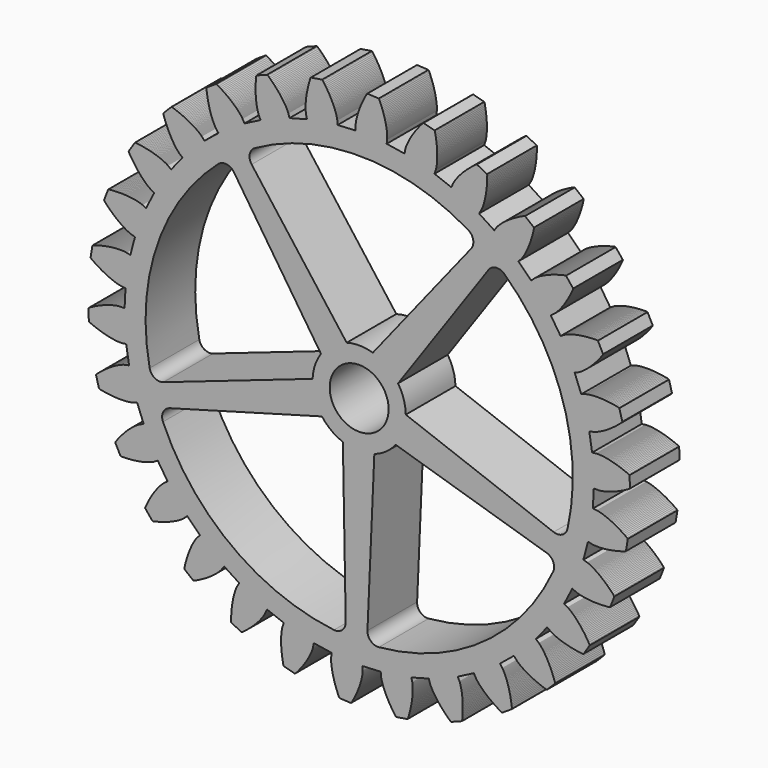
from build123d import *

# Parameters (mm, degrees)
F0_R     = 3.797782
F1_DEPTH = 8


# Not quite as in the source:
# - ends of sketch curves that miss each other by under 0.0002 mm in the source are joined


with BuildPart() as f1:
    # F0 (on Front) → F1 (new body)
    with BuildSketch(Plane.XZ):
        Polygon((-30.117293, 2.712268), (-30.236686, 0.387787), (-30.777096, 0.394663), (-30.78543, 0.394573), (-30.797925, 0.394291), (-30.814581, 0.393725), (-30.835394, 0.392777), (-30.86035, 0.391351), (-30.889447, 0.389347), (-30.92267, 0.386671), (-30.96001, 0.383226), (-31.001451, 0.378913), (-31.04698, 0.373644), (-31.096573, 0.367317), (-31.15022, 0.35984), (-31.207894, 0.351114), (-31.269576, 0.341048), (-31.335238, 0.329545), (-31.404858, 0.316515), (-31.478408, 0.301861), (-31.555862, 0.285489), (-31.637181, 0.26731), (-31.722344, 0.247231), (-31.811308, 0.225156), (-31.904043, 0.200998), (-32.000506, 0.174668), (-32.100667, 0.146072), (-32.204481, 0.115122), (-32.311902, 0.08173), (-32.422897, 0.045809), (-32.537413, 0.00727), (-32.655406, -0.033976), (-32.776828, -0.07801), (-32.901628, -0.12492), (-33.029758, -0.17479), (-33.161166, -0.227706), (-33.295794, -0.283746), (-33.433588, -0.342994), (-33.574489, -0.405532), (-33.718444, -0.471442), (-33.865391, -0.540798), (-34.015269, -0.613683), (-34.168013, -0.69017), (-34.323558, -0.770338), (-34.481844, -0.854264), (-34.6428, -0.942018), (-34.80636, -1.033678), (-34.915142, -1.127462), (-34.836389, -2.600837), (-34.718226, -2.682489), (-34.545831, -2.756192), (-34.376436, -2.826287), (-34.210107, -2.892861), (-34.046901, -2.955992), (-33.886875, -3.015765), (-33.730082, -3.072257), (-33.576582, -3.125552), (-33.426419, -3.175739), (-33.279653, -3.222902), (-33.136328, -3.267125), (-32.996493, -3.308494), (-32.860193, -3.347102), (-32.727478, -3.383027), (-32.598389, -3.416368), (-32.472965, -3.447208), (-32.351247, -3.475639), (-32.233276, -3.501753), (-32.119085, -3.52564), (-32.008712, -3.547388), (-31.902195, -3.567096), (-31.799556, -3.584851), (-31.700834, -3.600751), (-31.606052, -3.614884), (-31.515241, -3.627348), (-31.428425, -3.638238), (-31.345629, -3.647646), (-31.266877, -3.655665), (-31.192182, -3.662397), (-31.12157, -3.667931), (-31.055053, -3.67237), (-30.992651, -3.675804), (-30.934374, -3.67833), (-30.880239, -3.680046), (-30.830252, -3.68105), (-30.784423, -3.681442), (-30.742756, -3.681311), (-30.705264, -3.680754), (-30.671943, -3.679874), (-30.642798, -3.678764), (-30.617832, -3.677525), (-30.597037, -3.67625), (-30.580416, -3.675038), (-30.567963, -3.673983), (-30.559666, -3.673185), (-30.023068, -3.608741), (-29.656569, -5.907251), (-30.186598, -6.012883), (-30.194731, -6.014705), (-30.206896, -6.017575), (-30.223069, -6.021593), (-30.24323, -6.026847), (-30.267345, -6.033432), (-30.295389, -6.041444), (-30.327331, -6.050968), (-30.363138, -6.0621), (-30.402776, -6.074932), (-30.446213, -6.089552), (-30.493409, -6.106054), (-30.544327, -6.124522), (-30.598927, -6.145049), (-30.657167, -6.167716), (-30.719006, -6.192621), (-30.784395, -6.219842), (-30.853291, -6.249467), (-30.925647, -6.281584), (-31.00141, -6.316276), (-31.080535, -6.353622), (-31.162967, -6.393712), (-31.248651, -6.436619), (-31.337534, -6.482434), (-31.429559, -6.531227), (-31.52467, -6.583083), (-31.622805, -6.638081), (-31.723902, -6.696296), (-31.827901, -6.757801), (-31.934741, -6.822677), (-32.044356, -6.890995), (-32.156676, -6.962829), (-32.271639, -7.038248), (-32.389171, -7.117325), (-32.509204, -7.200134), (-32.63167, -7.286737), (-32.756491, -7.377204), (-32.8836, -7.471601), (-33.012915, -7.569996), (-33.144362, -7.672447), (-33.277866, -7.779019), (-33.413347, -7.889777), (-33.550722, -8.004778), (-33.689915, -8.12408), (-33.830841, -8.247742), (-33.91775, -8.362093), (-33.534386, -9.786899), (-33.401831, -9.842198), (-33.217875, -9.878447), (-33.03761, -9.911795), (-32.861075, -9.942331), (-32.68831, -9.97015), (-32.519351, -9.995342), (-32.354241, -10.018002), (-32.193013, -10.038218), (-32.035698, -10.056088), (-31.882334, -10.071706), (-31.732945, -10.085164), (-31.587564, -10.096556), (-31.446219, -10.105981), (-31.308935, -10.113529), (-31.175732, -10.119302), (-31.046637, -10.123391), (-30.921668, -10.125895), (-30.800844, -10.12691), (-30.684184, -10.126533), (-30.571702, -10.124861), (-30.463411, -10.121988), (-30.359328, -10.118017), (-30.259457, -10.113042), (-30.163809, -10.107162), (-30.072389, -10.100474), (-29.985208, -10.093073), (-29.902264, -10.085061), (-29.823564, -10.076532), (-29.749101, -10.067586), (-29.678882, -10.05832), (-29.612897, -10.04883), (-29.551143, -10.039216), (-29.493617, -10.029572), (-29.440304, -10.019994), (-29.391202, -10.010585), (-29.346292, -10.001433), (-29.305566, -9.992644), (-29.269008, -9.984306), (-29.236598, -9.976517), (-29.208323, -9.969373), (-29.184157, -9.962968), (-29.164084, -9.957396), (-29.148077, -9.952753), (-29.136115, -9.949134), (-29.128167, -9.946629), (-28.616692, -9.77203), (-27.780316, -11.94411), (-28.276802, -12.157635), (-28.284376, -12.161104), (-28.295679, -12.166445), (-28.310665, -12.173734), (-28.32929, -12.183066), (-28.351509, -12.194522), (-28.377274, -12.208187), (-28.40654, -12.224146), (-28.439249, -12.24248), (-28.475354, -12.263274), (-28.514803, -12.286605), (-28.557537, -12.312557), (-28.603499, -12.34121), (-28.652639, -12.372638), (-28.704893, -12.406921), (-28.760202, -12.444136), (-28.818503, -12.484359), (-28.879736, -12.527662), (-28.943833, -12.574122), (-29.010729, -12.623805), (-29.080359, -12.676786), (-29.152653, -12.733137), (-29.227546, -12.792923), (-29.304963, -12.856214), (-29.38483, -12.923076), (-29.467078, -12.993576), (-29.551635, -13.067774), (-29.63842, -13.145736), (-29.727361, -13.227522), (-29.818376, -13.313191), (-29.91139, -13.402805), (-30.006322, -13.496423), (-30.103092, -13.594095), (-30.201614, -13.695882), (-30.30181, -13.801836), (-30.403591, -13.912011), (-30.506877, -14.02645), (-30.611581, -14.145215), (-30.717611, -14.268342), (-30.824888, -14.395884), (-30.933315, -14.527888), (-31.042806, -14.664393), (-31.153272, -14.80544), (-31.264619, -14.951075), (-31.376755, -15.101334), (-31.437989, -15.231259), (-30.766769, -16.545219), (-30.625611, -16.571755), (-30.438141, -16.568964), (-30.254883, -16.564103), (-30.075854, -16.55727), (-29.901082, -16.548559), (-29.730578, -16.538074), (-29.564366, -16.525909), (-29.402457, -16.512163), (-29.244865, -16.496937), (-29.091602, -16.480325), (-28.942682, -16.462429), (-28.798109, -16.443348), (-28.657891, -16.423175), (-28.522037, -16.402017), (-28.390547, -16.379971), (-28.263422, -16.357128), (-28.140665, -16.333595), (-28.022269, -16.309468), (-27.908239, -16.284843), (-27.79856, -16.259821), (-27.693233, -16.234498), (-27.59225, -16.208972), (-27.495596, -16.183341), (-27.403258, -16.157704), (-27.315232, -16.132156), (-27.231492, -16.106792), (-27.152027, -16.081707), (-27.076817, -16.057004), (-27.005846, -16.032773), (-26.939084, -16.009107), (-26.876516, -15.986108), (-26.818111, -15.963862), (-26.763844, -15.942469), (-26.71369, -15.922016), (-26.667616, -15.902602), (-26.625593, -15.884318), (-26.587584, -15.86725), (-26.553558, -15.851493), (-26.523474, -15.837137), (-26.497303, -15.824267), (-26.474998, -15.812978), (-26.45652, -15.803357), (-26.441828, -15.795488), (-26.43088, -15.789461), (-26.423625, -15.785358), (-25.95963, -15.508231), (-24.68993, -17.458955), (-25.131172, -17.771036), (-25.137858, -17.776008), (-25.147804, -17.78358), (-25.160948, -17.793827), (-25.177226, -17.806827), (-25.196579, -17.822654), (-25.21894, -17.841377), (-25.244245, -17.863069), (-25.272428, -17.887806), (-25.303422, -17.915651), (-25.337156, -17.946674), (-25.373561, -17.980945), (-25.412564, -18.018526), (-25.454095, -18.059485), (-25.498078, -18.103883), (-25.544442, -18.151786), (-25.593107, -18.203251), (-25.643998, -18.258337), (-25.697034, -18.317107), (-25.75214, -18.379616), (-25.80923, -18.445915), (-25.86823, -18.516065), (-25.929055, -18.590115), (-25.99162, -18.668119), (-26.055842, -18.750127), (-26.121639, -18.836186), (-26.18892, -18.926343), (-26.2576, -19.020644), (-26.327591, -19.119135), (-26.398806, -19.221854), (-26.471157, -19.32885), (-26.544548, -19.440159), (-26.618897, -19.555818), (-26.694104, -19.675865), (-26.770078, -19.800333), (-26.846732, -19.92926), (-26.923967, -20.062677), (-27.00169, -20.200611), (-27.079805, -20.343095), (-27.158218, -20.490155), (-27.23683, -20.641817), (-27.315548, -20.798102), (-27.394273, -20.959035), (-27.47291, -21.124639), (-27.551356, -21.29493), (-27.584238, -21.434745), (-26.654497, -22.58044), (-26.510908, -22.577044), (-26.328115, -22.53534), (-26.149872, -22.492483), (-25.976178, -22.448575), (-25.807031, -22.403718), (-25.642436, -22.358013), (-25.482383, -22.311556), (-25.326869, -22.264447), (-25.175886, -22.216786), (-25.029428, -22.168674), (-24.887482, -22.120206), (-24.750039, -22.071484), (-24.617078, -22.022602), (-24.488591, -21.973661), (-24.364558, -21.924753), (-24.244961, -21.875982), (-24.129776, -21.827439), (-24.018988, -21.779224), (-23.912567, -21.73143), (-23.81049, -21.68415), (-23.71273, -21.637484), (-23.619258, -21.591518), (-23.530043, -21.546354), (-23.445058, -21.502078), (-23.364265, -21.458783), (-23.28763, -21.416565), (-23.215116, -21.37551), (-23.146686, -21.335705), (-23.082302, -21.297247), (-23.021919, -21.260222), (-22.965499, -21.224714), (-22.912998, -21.190814), (-22.864366, -21.158603), (-22.81956, -21.128174), (-22.778528, -21.099603), (-22.741225, -21.072978), (-22.707593, -21.048383), (-22.677588, -21.025893), (-22.651149, -21.005598), (-22.628223, -20.987571), (-22.608751, -20.971889), (-22.592679, -20.958637), (-22.579945, -20.947884), (-22.570489, -20.939713), (-22.564248, -20.934192), (-22.168008, -20.566649), (-20.520475, -22.210761), (-20.887189, -22.607763), (-20.892696, -22.614017), (-20.900852, -22.623489), (-20.911575, -22.636246), (-20.924794, -22.652345), (-20.940435, -22.671848), (-20.958416, -22.694813), (-20.978656, -22.721293), (-21.00108, -22.751347), (-21.025609, -22.785027), (-21.052156, -22.822388), (-21.08064, -22.863478), (-21.110978, -22.908346), (-21.143085, -22.957047), (-21.176875, -23.009621), (-21.212265, -23.066114), (-21.249167, -23.126571), (-21.287492, -23.191038), (-21.32715, -23.259549), (-21.368056, -23.332148), (-21.410118, -23.408869), (-21.453243, -23.489752), (-21.497341, -23.574832), (-21.54232, -23.664138), (-21.588089, -23.757705), (-21.634556, -23.855564), (-21.681622, -23.957738), (-21.729193, -24.064259), (-21.777179, -24.175147), (-21.825481, -24.290433), (-21.874003, -24.410131), (-21.922651, -24.534265), (-21.971327, -24.662857), (-22.019932, -24.795917), (-22.068368, -24.933463), (-22.116542, -25.075509), (-22.164347, -25.222067), (-22.211693, -25.373147), (-22.258478, -25.528758), (-22.304601, -25.688907), (-22.349966, -25.853599), (-22.39447, -26.022834), (-22.438016, -26.196622), (-22.4805, -26.374952), (-22.521828, -26.557834), (-22.524924, -26.701428), (-21.377296, -27.628784), (-21.237551, -27.59561), (-21.067422, -27.516811), (-20.901984, -27.43783), (-20.741215, -27.35877), (-20.585091, -27.279729), (-20.433593, -27.200799), (-20.2867, -27.122079), (-20.14438, -27.043669), (-20.006604, -26.965657), (-19.873351, -26.888147), (-19.744583, -26.811225), (-19.620272, -26.734989), (-19.500382, -26.659535), (-19.384876, -26.584948), (-19.273723, -26.511321), (-19.166879, -26.438752), (-19.064306, -26.367321), (-18.965959, -26.297125), (-18.871803, -26.228249), (-18.781785, -26.16078), (-18.695864, -26.094807), (-18.613991, -26.030414), (-18.53612, -25.967686), (-18.462194, -25.906708), (-18.392167, -25.847561), (-18.325983, -25.790333), (-18.263592, -25.735096), (-18.204934, -25.681938), (-18.149953, -25.630933), (-18.098587, -25.582161), (-18.050785, -25.535699), (-18.006475, -25.491622), (-17.965603, -25.450006), (-17.928105, -25.410925), (-17.893908, -25.374448), (-17.862956, -25.340648), (-17.835176, -25.309598), (-17.810498, -25.281364), (-17.788858, -25.256012), (-17.77018, -25.233613), (-17.754397, -25.214226), (-17.74143, -25.197921), (-17.73121, -25.184758), (-17.723657, -25.174797), (-17.718701, -25.1681), (-17.407539, -24.726208), (-15.454178, -25.991848), (-15.730336, -26.456421), (-15.734425, -26.463682), (-15.740428, -26.474642), (-15.748268, -26.489349), (-15.757852, -26.507846), (-15.769095, -26.530174), (-15.781906, -26.556375), (-15.796199, -26.586485), (-15.811886, -26.620547), (-15.828874, -26.65859), (-15.847074, -26.700654), (-15.866393, -26.746767), (-15.886738, -26.796965), (-15.90802, -26.851275), (-15.930144, -26.909723), (-15.953012, -26.972341), (-15.976537, -27.03915), (-16.000624, -27.110176), (-16.025171, -27.185435), (-16.050087, -27.26495), (-16.075278, -27.348743), (-16.100644, -27.436827), (-16.126089, -27.529213), (-16.15152, -27.62592), (-16.176834, -27.726959), (-16.201938, -27.83234), (-16.226734, -27.942068), (-16.25112, -28.05615), (-16.275, -28.174592), (-16.298277, -28.297401), (-16.320853, -28.424572), (-16.342627, -28.556109), (-16.363504, -28.692008), (-16.383382, -28.832265), (-16.402164, -28.976876), (-16.41975, -29.125836), (-16.436042, -29.279132), (-16.450941, -29.436754), (-16.464351, -29.598691), (-16.476171, -29.76493), (-16.4863, -29.935455), (-16.494647, -30.110247), (-16.501106, -30.289289), (-16.505586, -30.472558), (-16.507987, -30.660033), (-16.481161, -30.801135), (-15.165804, -31.46962), (-15.036009, -31.408114), (-14.885984, -31.295666), (-14.740578, -31.184016), (-14.599759, -31.073258), (-14.463485, -30.963482), (-14.331709, -30.85478), (-14.204389, -30.747238), (-14.081481, -30.64095), (-13.962936, -30.536001), (-13.84871, -30.432477), (-13.738751, -30.330467), (-13.633005, -30.230051), (-13.531424, -30.131317), (-13.433949, -30.034345), (-13.34053, -29.939218), (-13.251109, -29.846017), (-13.165631, -29.754823), (-13.084028, -29.665714), (-13.006248, -29.578767), (-12.932225, -29.494055), (-12.8619, -29.411661), (-12.795204, -29.331653), (-12.732075, -29.254105), (-12.672443, -29.17909), (-12.616244, -29.106677), (-12.563407, -29.036936), (-12.513861, -28.969938), (-12.467537, -28.905743), (-12.424362, -28.844421), (-12.384261, -28.786036), (-12.347159, -28.730652), (-12.312985, -28.678326), (-12.281659, -28.629124), (-12.253104, -28.583095), (-12.227241, -28.540308), (-12.203991, -28.500812), (-12.183273, -28.464663), (-12.165006, -28.431915), (-12.149109, -28.402619), (-12.135497, -28.376827), (-12.124089, -28.354584), (-12.114797, -28.335939), (-12.107536, -28.320936), (-12.102219, -28.309623), (-12.098762, -28.302043), (-11.886273, -27.805112), (-9.712457, -28.636969), (-9.885991, -29.148803), (-9.888481, -29.156756), (-9.892077, -29.168727), (-9.896684, -29.184743), (-9.902215, -29.204828), (-9.908568, -29.229007), (-9.915652, -29.257299), (-9.923375, -29.289724), (-9.931636, -29.326301), (-9.940343, -29.367045), (-9.949399, -29.41197), (-9.958709, -29.461095), (-9.968174, -29.514426), (-9.977699, -29.571974), (-9.987184, -29.633745), (-9.996536, -29.69975), (-10.005658, -29.769989), (-10.014448, -29.844467), (-10.022813, -29.923189), (-10.030654, -30.006149), (-10.037871, -30.093346), (-10.044369, -30.184777), (-10.05005, -30.280437), (-10.054819, -30.380318), (-10.058572, -30.484413), (-10.061218, -30.592709), (-10.062657, -30.705193), (-10.062791, -30.821853), (-10.061524, -30.942674), (-10.058761, -31.067638), (-10.054403, -31.196723), (-10.048355, -31.329914), (-10.040519, -31.467183), (-10.030803, -31.608508), (-10.019107, -31.753864), (-10.005337, -31.903226), (-9.989401, -32.056555), (-9.971203, -32.213835), (-9.950652, -32.375019), (-9.927651, -32.540083), (-9.902105, -32.708989), (-9.873925, -32.881695), (-9.843023, -33.058166), (-9.8093, -33.238362), (-9.772669, -33.422241), (-9.717093, -33.554681), (-8.291494, -33.935079), (-8.177324, -33.847934), (-8.053955, -33.70675), (-7.934941, -33.567309), (-7.820229, -33.429692), (-7.709752, -33.293984), (-7.603458, -33.160258), (-7.501278, -33.028596), (-7.403157, -32.899076), (-7.309024, -32.771775), (-7.218815, -32.646765), (-7.132468, -32.52412), (-7.049909, -32.403912), (-6.971077, -32.286217), (-6.895894, -32.171096), (-6.824295, -32.058628), (-6.756206, -31.948872), (-6.691553, -31.841899), (-6.630264, -31.737768), (-6.572261, -31.63655), (-6.517467, -31.538303), (-6.465809, -31.443086), (-6.417205, -31.350957), (-6.371579, -31.261979), (-6.328847, -31.176205), (-6.288931, -31.093692), (-6.251747, -31.014491), (-6.217216, -30.938653), (-6.185251, -30.866231), (-6.155766, -30.797271), (-6.128682, -30.731825), (-6.103907, -30.669935), (-6.081359, -30.61165), (-6.060948, -30.557008), (-6.042585, -30.506051), (-6.026183, -30.458819), (-6.011653, -30.415353), (-5.998901, -30.375689), (-5.987843, -30.339859), (-5.978384, -30.307895), (-5.970435, -30.279837), (-5.963899, -30.255706), (-5.958685, -30.235535), (-5.954704, -30.219354), (-5.951856, -30.207184), (-5.950052, -30.199048), (-5.845524, -29.668799), (-3.546256, -30.030514), (-3.609582, -30.567246), (-3.610363, -30.575542), (-3.611391, -30.587998), (-3.61257, -30.604624), (-3.6138, -30.62542), (-3.614992, -30.650388), (-3.61604, -30.679535), (-3.616851, -30.712857), (-3.617328, -30.750352), (-3.617371, -30.792017), (-3.616888, -30.837847), (-3.61578, -30.887832), (-3.613952, -30.941963), (-3.611303, -31.000234), (-3.607737, -31.062628), (-3.603163, -31.129136), (-3.597482, -31.199738), (-3.590596, -31.274417), (-3.582409, -31.353155), (-3.572829, -31.435933), (-3.561761, -31.522725), (-3.549107, -31.613508), (-3.534778, -31.708258), (-3.518675, -31.806949), (-3.500703, -31.909548), (-3.480776, -32.016027), (-3.458795, -32.126355), (-3.434673, -32.240493), (-3.408313, -32.35841), (-3.379629, -32.480068), (-3.348527, -32.605428), (-3.31492, -32.734449), (-3.278716, -32.86709), (-3.239827, -33.003306), (-3.198166, -33.143056), (-3.153645, -33.286288), (-3.106178, -33.432957), (-3.055678, -33.583013), (-3.002061, -33.736404), (-2.945243, -33.893078), (-2.885139, -34.052981), (-2.821669, -34.216055), (-2.754748, -34.382246), (-2.684299, -34.551495), (-2.61024, -34.723738), (-2.528339, -34.841729), (-1.054806, -34.917417), (-0.961249, -34.808436), (-0.86993, -34.644688), (-0.78251, -34.483549), (-0.698914, -34.325089), (-0.619067, -34.169375), (-0.542898, -34.016473), (-0.470327, -33.866447), (-0.401277, -33.719356), (-0.335667, -33.575263), (-0.273422, -33.434229), (-0.214461, -33.296314), (-0.158701, -33.161567), (-0.106061, -33.030052), (-0.056456, -32.901819), (-0.009806, -32.776919), (0.033977, -32.655408), (0.074975, -32.53733), (0.113278, -32.422731), (0.148968, -32.311666), (0.182137, -32.204171), (0.212868, -32.100294), (0.241256, -32.000078), (0.267386, -31.903557), (0.291352, -31.810771), (0.313239, -31.721761), (0.333142, -31.636561), (0.351151, -31.555199), (0.367362, -31.477714), (0.381865, -31.404135), (0.394749, -31.334487), (0.406115, -31.2688), (0.416054, -31.207097), (0.424658, -31.149406), (0.432024, -31.095746), (0.438248, -31.046137), (0.443424, -31.000598), (0.447647, -30.959148), (0.451015, -30.921801), (0.453622, -30.888571), (0.455568, -30.859472), (0.456942, -30.834509), (0.457848, -30.813697), (0.458379, -30.797042), (0.458631, -30.784544), (0.458705, -30.776213), (0.450704, -30.235818), (2.774932, -30.111584), (2.824581, -30.649751), (2.825542, -30.65803), (2.827129, -30.670428), (2.829433, -30.686935), (2.832552, -30.707531), (2.836579, -30.732203), (2.841614, -30.760933), (2.847748, -30.793692), (2.855078, -30.830469), (2.863697, -30.871232), (2.873696, -30.91596), (2.885174, -30.96462), (2.898216, -31.017192), (2.912922, -31.073637), (2.929383, -31.133929), (2.947686, -31.198028), (2.967921, -31.265906), (2.990185, -31.337524), (3.014563, -31.412837), (3.041141, -31.491813), (3.070014, -31.574409), (3.101266, -31.66058), (3.134984, -31.75028), (3.171254, -31.843464), (3.210163, -31.940086), (3.251793, -32.040096), (3.29623, -32.143441), (3.343559, -32.250072), (3.393857, -32.359931), (3.447209, -32.472967), (3.503695, -32.589118), (3.563394, -32.708334), (3.626385, -32.830549), (3.692745, -32.955704), (3.76255, -33.083738), (3.835879, -33.214582), (3.912802, -33.348178), (3.993397, -33.484454), (4.077733, -33.623346), (4.165884, -33.764783), (4.257921, -33.908696), (4.353909, -34.055012), (4.453919, -34.203655), (4.558018, -34.354559), (4.666271, -34.507638), (4.770911, -34.606023), (6.227983, -34.373693), (6.296838, -34.247643), (6.352116, -34.068487), (6.404122, -33.892693), (6.452947, -33.720316), (6.498671, -33.551407), (6.541389, -33.386007), (6.581179, -33.224169), (6.618139, -33.065936), (6.652357, -32.911353), (6.68392, -32.76046), (6.712917, -32.613297), (6.739445, -32.469906), (6.763592, -32.330319), (6.78545, -32.194574), (6.805113, -32.062705), (6.822675, -31.934743), (6.838228, -31.810721), (6.851866, -31.690667), (6.863685, -31.574606), (6.873779, -31.462567), (6.882245, -31.354569), (6.889175, -31.250638), (6.894664, -31.150793), (6.898814, -31.055055), (6.901718, -30.96344), (6.903472, -30.87596), (6.904174, -30.792633), (6.903918, -30.713473), (6.902804, -30.638485), (6.900931, -30.567679), (6.898389, -30.501063), (6.895282, -30.438646), (6.891702, -30.380425), (6.887754, -30.326404), (6.883526, -30.276586), (6.879122, -30.230967), (6.874633, -30.189546), (6.870165, -30.152314), (6.865803, -30.11927), (6.861657, -30.090401), (6.857811, -30.065699), (6.85437, -30.045154), (6.851426, -30.02875), (6.849075, -30.016474), (6.847417, -30.008307), (6.727235, -29.481386), (8.974844, -28.876634), (9.1353, -29.392719), (9.13796, -29.400614), (9.142089, -29.412412), (9.147774, -29.428078), (9.155106, -29.447578), (9.164178, -29.470874), (9.175075, -29.497926), (9.187886, -29.528698), (9.202701, -29.563144), (9.219607, -29.601226), (9.238688, -29.642897), (9.26003, -29.688107), (9.283721, -29.736816), (9.30984, -29.788972), (9.338474, -29.844525), (9.369705, -29.903418), (9.403612, -29.965605), (9.440279, -30.031027), (9.479783, -30.09963), (9.522201, -30.171352), (9.567617, -30.246139), (9.616099, -30.323929), (9.66773, -30.404659), (9.722582, -30.488266), (9.78073, -30.57469), (9.842243, -30.663855), (9.907199, -30.755705), (9.975659, -30.850164), (10.047703, -30.947164), (10.123389, -31.046639), (10.202788, -31.148509), (10.285971, -31.252708), (10.372995, -31.359157), (10.463925, -31.467778), (10.558824, -31.5785), (10.657756, -31.69124), (10.760776, -31.805925), (10.867941, -31.922467), (10.979313, -32.040787), (11.094943, -32.160805), (11.214889, -32.282438), (11.339201, -32.4056), (11.467929, -32.530201), (11.601127, -32.656164), (11.738842, -32.783392), (11.861653, -32.857872), (13.23858, -32.327673), (13.279723, -32.190063), (13.296542, -32.003329), (13.310864, -31.820566), (13.322783, -31.641804), (13.33239, -31.467077), (13.339783, -31.296413), (13.34506, -31.129838), (13.348313, -30.967377), (13.349642, -30.809058), (13.34914, -30.654901), (13.346911, -30.504924), (13.343045, -30.359151), (13.337642, -30.217593), (13.330799, -30.080271), (13.322614, -29.947194), (13.313189, -29.818378), (13.302616, -29.693834), (13.290995, -29.573565), (13.278428, -29.457583), (13.265004, -29.345895), (13.25083, -29.238497), (13.236002, -29.135398), (13.220615, -29.036592), (13.204769, -28.942084), (13.188561, -28.851865), (13.172088, -28.765933), (13.155448, -28.684284), (13.138741, -28.606904), (13.122061, -28.533786), (13.105504, -28.464917), (13.08917, -28.400287), (13.073153, -28.339878), (13.05755, -28.283675), (13.042453, -28.231656), (13.027961, -28.183805), (13.014166, -28.1401), (13.001166, -28.100516), (12.989051, -28.065027), (12.977918, -28.033611), (12.967858, -28.006236), (12.958963, -27.982874), (12.951325, -27.963491), (12.945035, -27.948059), (12.940185, -27.936537), (12.93686, -27.928895), (12.709754, -27.438475), (14.782512, -26.379634), (15.046761, -26.851082), (15.051005, -26.858253), (15.057497, -26.868935), (15.066316, -26.883076), (15.077542, -26.900625), (15.091256, -26.921524), (15.107541, -26.945721), (15.126471, -26.973155), (15.148124, -27.003768), (15.172577, -27.037502), (15.199906, -27.074297), (15.230183, -27.114083), (15.263482, -27.156804), (15.299875, -27.202388), (15.339432, -27.250773), (15.382226, -27.301885), (15.42832, -27.355664), (15.477788, -27.412033), (15.530691, -27.470923), (15.587094, -27.532259), (15.647066, -27.595972), (15.710664, -27.661979), (15.77795, -27.730211), (15.848989, -27.800587), (15.923833, -27.873029), (16.00254, -27.947461), (16.085172, -28.023796), (16.171776, -28.101957), (16.262413, -28.181861), (16.357126, -28.263424), (16.455972, -28.34656), (16.559001, -28.431188), (16.666254, -28.517217), (16.777783, -28.60456), (16.89363, -28.693129), (17.013838, -28.782838), (17.138448, -28.873595), (17.267503, -28.96531), (17.40104, -29.057892), (17.539098, -29.151246), (17.681712, -29.245284), (17.828914, -29.339908), (17.980738, -29.435023), (18.137214, -29.530535), (18.298373, -29.626354), (18.433981, -29.673671), (19.670585, -28.868781), (19.68222, -28.725624), (19.659847, -28.539472), (19.635858, -28.357724), (19.610348, -28.180392), (19.583419, -28.007485), (19.555165, -27.839013), (19.525695, -27.674983), (19.495101, -27.515396), (19.463483, -27.360261), (19.430943, -27.209574), (19.397577, -27.063341), (19.363488, -26.921556), (19.328773, -26.784214), (19.293529, -26.651314), (19.257855, -26.522849), (19.221852, -26.398808), (19.185616, -26.279182), (19.149245, -26.16396), (19.112837, -26.053126), (19.076487, -25.946666), (19.040295, -25.844564), (19.004352, -25.746798), (18.968759, -25.653353), (18.933609, -25.564204), (18.898997, -25.479327), (18.865019, -25.3987), (18.831769, -25.322291), (18.799336, -25.250077), (18.76782, -25.182026), (18.737308, -25.118104), (18.707891, -25.058281), (18.679666, -25.002524), (18.652715, -24.950789), (18.627135, -24.903048), (18.603011, -24.859257), (18.580432, -24.819372), (18.559483, -24.783357), (18.540258, -24.751164), (18.522834, -24.722747), (18.507302, -24.698062), (18.493743, -24.67706), (18.482244, -24.659691), (18.472883, -24.6459), (18.46574, -24.635642), (18.460904, -24.628856), (18.136795, -24.196373), (19.944112, -22.72972), (20.300607, -23.135922), (20.30625, -23.142053), (20.314819, -23.151154), (20.326384, -23.163152), (20.341015, -23.177983), (20.358777, -23.195577), (20.379734, -23.215857), (20.403956, -23.238758), (20.431499, -23.264199), (20.462433, -23.292112), (20.496814, -23.32242), (20.5347, -23.355043), (20.576153, -23.389906), (20.621228, -23.426928), (20.669983, -23.466031), (20.722466, -23.507131), (20.778737, -23.550149), (20.838843, -23.595002), (20.902834, -23.641604), (20.970759, -23.689875), (21.042664, -23.739723), (21.118598, -23.791067), (21.198601, -23.84382), (21.282717, -23.897889), (21.370987, -23.953188), (21.463452, -24.009624), (21.560147, -24.067114), (21.661111, -24.125562), (21.766377, -24.184875), (21.87598, -24.244963), (21.989953, -24.30573), (22.10832, -24.367088), (22.23112, -24.428937), (22.358368, -24.491185), (22.4901, -24.553735), (22.626332, -24.616491), (22.767089, -24.679357), (22.912393, -24.742235), (23.062263, -24.805028), (23.216711, -24.867638), (23.375761, -24.929969), (23.539418, -24.99192), (23.707699, -25.05339), (23.880616, -25.114284), (24.058172, -25.174501), (24.20066, -25.19259), (25.242892, -24.148185), (25.224507, -24.005737), (25.163924, -23.828305), (25.102668, -23.655516), (25.040846, -23.487363), (24.978558, -23.323836), (24.915896, -23.164918), (24.852963, -23.010596), (24.789856, -22.86086), (24.726678, -22.715686), (24.663519, -22.575061), (24.60048, -22.438958), (24.537655, -22.307357), (24.475142, -22.180238), (24.413038, -22.057569), (24.351436, -21.939328), (24.29043, -21.825483), (24.230115, -21.716006), (24.170583, -21.610863), (24.111926, -21.510019), (24.054236, -21.413445), (23.997605, -21.321099), (23.942123, -21.232941), (23.887877, -21.148939), (23.834962, -21.069045), (23.783461, -20.99322), (23.733461, -20.921417), (23.685048, -20.853594), (23.638314, -20.7897), (23.593335, -20.729687), (23.550199, -20.673506), (23.50899, -20.621107), (23.469784, -20.572435), (23.432669, -20.527438), (23.397722, -20.486059), (23.365019, -20.44824), (23.334642, -20.413921), (23.306664, -20.383047), (23.281165, -20.355555), (23.258214, -20.331384), (23.237888, -20.310466), (23.220258, -20.29274), (23.205399, -20.278142), (23.193376, -20.266603), (23.184259, -20.258052), (23.178115, -20.252421), (22.771171, -19.896771), (24.23406, -18.086406), (24.667219, -18.409613), (24.674013, -18.41444), (24.684288, -18.421558), (24.698094, -18.430889), (24.71549, -18.442353), (24.73652, -18.455868), (24.761237, -18.471349), (24.789689, -18.488713), (24.821921, -18.507874), (24.857983, -18.528745), (24.897911, -18.55124), (24.941754, -18.575276), (24.98955, -18.600755), (25.041339, -18.627599), (25.097155, -18.655709), (25.157038, -18.685001), (25.221024, -18.715378), (25.28914, -18.746754), (25.361421, -18.779035), (25.4379, -18.81213), (25.518598, -18.845937), (25.603546, -18.880372), (25.692768, -18.915337), (25.786288, -18.950737), (25.884127, -18.986474), (25.986303, -19.022456), (26.092839, -19.058583), (26.203747, -19.094762), (26.319048, -19.130894), (26.43875, -19.166881), (26.562863, -19.202624), (26.691402, -19.238031), (26.824375, -19.272997), (26.961787, -19.307427), (27.103644, -19.341222), (27.249949, -19.374283), (27.400699, -19.406509), (27.555903, -19.437803), (27.715551, -19.468064), (27.879645, -19.497196), (28.048176, -19.525095), (28.221137, -19.551668), (28.398524, -19.576807), (28.580319, -19.600418), (28.766518, -19.622402), (28.90965, -19.610472), (29.711966, -18.372196), (29.664365, -18.236684), (29.568214, -18.075725), (29.472373, -17.919448), (29.37694, -17.767824), (29.282012, -17.620818), (29.18768, -17.478401), (29.094039, -17.340539), (29.001179, -17.207195), (28.909195, -17.078329), (28.818179, -16.953906), (28.728221, -16.833886), (28.639408, -16.718224), (28.551834, -16.606879), (28.465581, -16.499804), (28.38074, -16.396954), (28.297399, -16.298278), (28.215639, -16.203734), (28.135547, -16.113266), (28.057207, -16.026822), (27.980696, -15.944352), (27.906104, -15.865798), (27.833506, -15.791105), (27.762982, -15.720214), (27.69461, -15.653069), (27.628471, -15.58961), (27.564634, -15.529771), (27.503181, -15.473494), (27.444179, -15.420712), (27.387708, -15.371364), (27.333836, -15.325382), (27.282631, -15.282694), (27.234165, -15.243237), (27.188505, -15.206938), (27.145717, -15.173729), (27.105864, -15.143534), (27.069017, -15.116282), (27.035231, -15.0919), (27.004573, -15.07031), (26.977099, -15.051439), (26.952867, -15.035204), (26.93194, -15.021533), (26.914368, -15.010342), (26.900207, -15.001553), (26.889511, -14.995085), (26.882333, -14.990856), (26.410337, -14.727586), (27.464862, -12.652631), (27.955752, -12.878717), (27.963404, -12.882022), (27.974933, -12.88685), (27.990377, -12.893107), (28.009778, -12.900706), (28.033158, -12.909554), (28.060555, -12.919557), (28.091993, -12.930625), (28.127506, -12.942665), (28.167119, -12.955583), (28.210851, -12.969284), (28.258735, -12.983677), (28.310783, -12.998665), (28.36702, -13.014154), (28.427462, -13.030044), (28.492127, -13.046245), (28.561028, -13.06266), (28.634182, -13.079185), (28.711594, -13.095732), (28.793281, -13.112203), (28.879244, -13.128496), (28.969498, -13.144517), (29.064038, -13.160167), (29.162874, -13.175347), (29.266005, -13.189961), (29.373432, -13.203913), (29.48515, -13.2171), (29.601159, -13.229429), (29.721448, -13.240798), (29.846015, -13.251111), (29.974852, -13.26027), (30.107942, -13.268177), (30.245279, -13.274734), (30.386849, -13.279841), (30.532631, -13.283404), (30.682611, -13.285324), (30.836769, -13.285503), (30.995087, -13.283845), (31.157538, -13.280253), (31.324102, -13.27463), (31.494751, -13.266881), (31.669457, -13.256912), (31.848192, -13.244622), (32.030928, -13.229922), (32.217626, -13.21271), (32.355149, -13.17128), (32.88248, -11.793255), (32.807746, -11.670601), (32.680231, -11.53315), (32.553994, -11.400215), (32.429121, -11.271743), (32.305705, -11.147688), (32.183821, -11.027996), (32.063562, -10.912615), (31.945011, -10.801491), (31.828243, -10.694569), (31.713348, -10.591788), (31.600402, -10.493093), (31.489481, -10.398424), (31.380671, -10.307718), (31.274041, -10.220915), (31.16967, -10.137954), (31.067636, -10.058763), (30.968004, -9.983283), (30.870854, -9.911442), (30.776252, -9.843178), (30.684268, -9.778415), (30.594972, -9.717087), (30.508433, -9.659122), (30.42471, -9.604442), (30.343872, -9.552979), (30.265983, -9.504655), (30.191102, -9.4594), (30.11929, -9.417129), (30.050604, -9.377767), (29.985106, -9.34124), (29.92285, -9.307459), (29.863888, -9.276354), (29.80828, -9.247834), (29.756068, -9.221824), (29.70731, -9.198236), (29.662053, -9.176985), (29.620344, -9.157991), (29.582229, -9.141165), (29.54775, -9.126423), (29.516952, -9.113673), (29.489877, -9.102832), (29.466564, -9.093811), (29.447049, -9.086519), (29.431371, -9.080868), (29.419564, -9.076763), (29.411662, -9.074117), (28.895243, -8.914735), (29.495318, -6.665875), (30.022489, -6.784958), (30.030659, -6.786602), (30.042941, -6.788925), (30.059349, -6.791834), (30.079903, -6.795235), (30.104612, -6.799027), (30.13349, -6.803115), (30.166545, -6.807407), (30.203784, -6.811799), (30.245216, -6.816201), (30.290844, -6.820511), (30.34067, -6.824634), (30.394699, -6.828472), (30.452925, -6.831927), (30.515353, -6.834906), (30.58197, -6.837309), (30.652779, -6.839036), (30.72777, -6.839995), (30.806933, -6.840083), (30.890257, -6.839209), (30.977731, -6.837272), (31.069341, -6.834179), (31.165071, -6.829829), (31.264905, -6.82413), (31.36882, -6.816983), (31.476799, -6.808297), (31.588818, -6.797968), (31.704855, -6.785907), (31.824882, -6.77202), (31.94887, -6.756208), (32.076795, -6.738381), (32.208621, -6.718442), (32.344321, -6.696302), (32.483857, -6.671866), (32.627193, -6.64504), (32.774294, -6.615736), (32.925123, -6.583859), (33.079634, -6.549322), (33.237791, -6.512031), (33.399544, -6.471903), (33.564855, -6.428841), (33.733671, -6.382765), (33.905945, -6.333585), (34.081628, -6.28121), (34.26067, -6.22556), (34.386577, -6.156442), (34.615876, -4.698891), (34.517271, -4.594455), (34.363967, -4.486521), (34.212848, -4.382735), (34.063994, -4.283036), (33.917481, -4.18735), (33.773379, -4.095616), (33.631757, -4.007761), (33.492692, -3.923713), (33.356246, -3.843402), (33.222491, -3.766755), (33.091494, -3.6937), (32.963314, -3.62416), (32.838021, -3.55806), (32.715675, -3.495325), (32.596337, -3.435875), (32.480065, -3.379631), (32.366921, -3.326512), (32.256958, -3.276445), (32.150228, -3.22934), (32.046792, -3.185117), (31.946694, -3.143692), (31.849993, -3.104986), (31.756731, -3.068908), (31.666963, -3.035377), (31.580728, -3.004306), (31.498071, -2.975606), (31.41904, -2.949189), (31.343676, -2.924968), (31.272011, -2.902855), (31.204094, -2.882758), (31.139955, -2.86459), (31.079628, -2.848258), (31.023153, -2.83367), (30.970557, -2.820733), (30.921869, -2.809359), (30.877122, -2.799451), (30.836339, -2.79092), (30.799549, -2.783665), (30.766776, -2.777598), (30.738037, -2.772624), (30.713357, -2.768646), (30.692752, -2.765571), (30.676244, -2.763303), (30.663841, -2.761742), (30.655561, -2.760797), (30.117293, -2.712269), (30.236686, -0.387788), (30.777096, -0.394663), (30.78543, -0.394573), (30.797925, -0.394292), (30.814581, -0.393726), (30.835394, -0.392778), (30.86035, -0.391352), (30.889447, -0.389347), (30.92267, -0.386672), (30.96001, -0.383227), (31.001451, -0.378914), (31.04698, -0.373645), (31.096573, -0.367318), (31.150219, -0.359841), (31.207894, -0.351115), (31.269575, -0.341048), (31.335238, -0.329546), (31.404857, -0.316516), (31.478408, -0.301862), (31.555862, -0.28549), (31.637181, -0.26731), (31.722343, -0.247231), (31.811308, -0.225157), (31.904042, -0.200999), (32.000506, -0.174668), (32.100667, -0.146072), (32.204481, -0.115123), (32.311902, -0.08173), (32.422897, -0.045809), (32.537413, -0.00727), (32.655406, 0.033975), (32.776828, 0.07801), (32.901628, 0.124919), (33.029758, 0.174789), (33.161165, 0.227706), (33.295794, 0.283745), (33.433587, 0.342993), (33.574489, 0.405532), (33.718444, 0.471441), (33.865391, 0.540797), (34.015269, 0.613682), (34.168012, 0.690169), (34.323558, 0.770338), (34.481844, 0.854264), (34.6428, 0.942017), (34.80636, 1.033677), (34.915142, 1.127462), (34.836389, 2.600837), (34.718226, 2.682488), (34.545831, 2.756192), (34.376436, 2.826287), (34.210107, 2.892861), (34.046901, 2.955992), (33.886874, 3.015764), (33.730081, 3.072256), (33.576582, 3.125551), (33.426419, 3.175738), (33.279653, 3.222901), (33.136327, 3.267125), (32.996493, 3.308493), (32.860193, 3.347101), (32.727478, 3.383026), (32.598389, 3.416367), (32.472965, 3.447207), (32.351247, 3.475639), (32.233276, 3.501752), (32.119085, 3.525639), (32.008712, 3.547388), (31.902195, 3.567095), (31.799556, 3.58485), (31.700833, 3.60075), (31.606051, 3.614883), (31.515241, 3.627348), (31.428425, 3.638238), (31.345629, 3.647645), (31.266877, 3.655664), (31.192182, 3.662396), (31.121569, 3.66793), (31.055053, 3.672369), (30.992651, 3.675803), (30.934374, 3.678329), (30.880239, 3.680045), (30.830252, 3.68105), (30.784423, 3.681441), (30.742756, 3.68131), (30.705264, 3.680753), (30.671943, 3.679874), (30.642798, 3.678764), (30.617831, 3.677525), (30.597037, 3.676249), (30.580416, 3.675037), (30.567963, 3.673982), (30.559666, 3.673184), (30.023067, 3.608741), (29.656569, 5.90725), (30.186598, 6.012883), (30.194731, 6.014704), (30.206896, 6.017575), (30.223069, 6.021592), (30.24323, 6.026846), (30.267345, 6.033431), (30.295389, 6.041443), (30.32733, 6.050967), (30.363138, 6.062099), (30.402776, 6.074931), (30.446213, 6.089552), (30.493409, 6.106053), (30.544327, 6.124521), (30.598927, 6.145048), (30.657167, 6.167716), (30.719006, 6.192621), (30.784395, 6.219841), (30.853291, 6.249467), (30.925647, 6.281583), (31.00141, 6.316276), (31.080535, 6.353621), (31.162967, 6.393711), (31.248651, 6.436619), (31.337533, 6.482433), (31.429559, 6.531227), (31.52467, 6.583083), (31.622804, 6.63808), (31.723902, 6.696295), (31.827901, 6.757801), (31.934741, 6.822676), (32.044356, 6.890994), (32.156676, 6.962828), (32.271638, 7.038247), (32.38917, 7.117325), (32.509203, 7.200133), (32.631669, 7.286736), (32.756491, 7.377203), (32.883599, 7.471601), (33.012915, 7.569995), (33.144362, 7.672447), (33.277866, 7.779018), (33.413346, 7.889776), (33.550722, 8.004778), (33.689915, 8.124079), (33.830841, 8.247741), (33.917749, 8.362093), (33.534386, 9.786898), (33.401831, 9.842198), (33.217875, 9.878446), (33.03761, 9.911795), (32.861074, 9.942331), (32.68831, 9.970149), (32.519351, 9.995341), (32.35424, 10.018001), (32.193012, 10.038217), (32.035698, 10.056087), (31.882334, 10.071706), (31.732945, 10.085164), (31.587564, 10.096556), (31.446219, 10.10598), (31.308935, 10.113528), (31.175732, 10.119301), (31.046637, 10.12339), (30.921668, 10.125894), (30.800844, 10.12691), (30.684183, 10.126532), (30.571702, 10.12486), (30.463411, 10.121988), (30.359328, 10.118017), (30.259457, 10.113042), (30.163809, 10.107161), (30.072389, 10.100473), (29.985208, 10.093072), (29.902264, 10.08506), (29.823564, 10.076532), (29.749101, 10.067586), (29.678881, 10.05832), (29.612897, 10.048829), (29.551143, 10.039216), (29.493617, 10.029571), (29.440304, 10.019993), (29.391202, 10.010584), (29.346292, 10.001433), (29.305566, 9.992643), (29.269008, 9.984305), (29.236598, 9.976516), (29.208322, 9.969372), (29.184157, 9.962968), (29.164084, 9.957395), (29.148077, 9.952753), (29.136115, 9.949133), (29.128167, 9.946628), (28.616692, 9.772029), (27.780316, 11.94411), (28.276802, 12.157634), (28.284376, 12.161104), (28.295679, 12.166445), (28.310665, 12.173733), (28.32929, 12.183065), (28.351509, 12.194522), (28.377274, 12.208187), (28.40654, 12.224145), (28.439249, 12.24248), (28.475354, 12.263273), (28.514802, 12.286605), (28.557537, 12.312557), (28.603499, 12.341209), (28.652638, 12.372637), (28.704893, 12.406921), (28.760202, 12.444136), (28.818503, 12.484358), (28.879736, 12.527661), (28.943833, 12.574121), (29.010729, 12.623804), (29.080359, 12.676786), (29.152653, 12.733137), (29.227546, 12.792922), (29.304963, 12.856213), (29.38483, 12.923076), (29.467078, 12.993576), (29.551634, 13.067773), (29.63842, 13.145735), (29.727361, 13.227521), (29.818376, 13.313191), (29.91139, 13.402805), (30.006322, 13.496423), (30.103091, 13.594095), (30.201613, 13.695881), (30.30181, 13.801835), (30.40359, 13.91201), (30.506876, 14.02645), (30.611581, 14.145214), (30.717611, 14.268341), (30.824887, 14.395883), (30.933315, 14.527888), (31.042806, 14.664392), (31.153272, 14.80544), (31.264619, 14.951075), (31.376755, 15.101334), (31.437989, 15.231258), (30.766768, 16.545219), (30.625611, 16.571754), (30.438141, 16.568964), (30.254883, 16.564102), (30.075854, 16.55727), (29.901082, 16.548559), (29.730578, 16.538074), (29.564366, 16.525909), (29.402457, 16.512162), (29.244865, 16.496936), (29.091602, 16.480324), (28.942681, 16.462428), (28.798109, 16.443347), (28.657891, 16.423175), (28.522037, 16.402017), (28.390547, 16.37997), (28.263422, 16.357128), (28.140665, 16.333594), (28.022269, 16.309467), (27.908239, 16.284842), (27.79856, 16.25982), (27.693233, 16.234497), (27.59225, 16.208971), (27.495596, 16.183341), (27.403258, 16.157704), (27.315232, 16.132156), (27.231492, 16.106792), (27.152026, 16.081707), (27.076817, 16.057003), (27.005846, 16.032772), (26.939084, 16.009107), (26.876516, 15.986108), (26.818111, 15.963861), (26.763844, 15.942469), (26.71369, 15.922016), (26.667616, 15.902601), (26.625593, 15.884317), (26.587584, 15.867249), (26.553558, 15.851493), (26.523474, 15.837137), (26.497303, 15.824266), (26.474998, 15.812978), (26.45652, 15.803356), (26.441827, 15.795487), (26.43088, 15.78946), (26.423625, 15.785358), (25.95963, 15.50823), (24.68993, 17.458954), (25.131171, 17.771036), (25.137858, 17.776007), (25.147804, 17.78358), (25.160948, 17.793826), (25.177226, 17.806827), (25.196579, 17.822654), (25.21894, 17.841376), (25.244245, 17.863068), (25.272428, 17.887805), (25.303422, 17.91565), (25.337156, 17.946673), (25.373561, 17.980944), (25.412563, 18.018525), (25.454095, 18.059484), (25.498078, 18.103883), (25.544442, 18.151785), (25.593107, 18.203251), (25.643997, 18.258337), (25.697034, 18.317106), (25.75214, 18.379615), (25.80923, 18.445915), (25.868229, 18.516064), (25.929054, 18.590114), (25.99162, 18.668118), (26.055842, 18.750126), (26.121639, 18.836185), (26.188919, 18.926342), (26.257599, 19.020644), (26.327591, 19.119134), (26.398806, 19.221854), (26.471156, 19.328849), (26.544548, 19.440158), (26.618896, 19.555817), (26.694103, 19.675864), (26.770078, 19.800333), (26.846732, 19.92926), (26.923967, 20.062677), (27.00169, 20.20061), (27.079805, 20.343095), (27.158217, 20.490154), (27.23683, 20.641816), (27.315548, 20.798101), (27.394273, 20.959034), (27.47291, 21.124639), (27.551356, 21.294929), (27.584238, 21.434745), (26.654497, 22.580439), (26.510908, 22.577044), (26.328114, 22.535339), (26.149872, 22.492482), (25.976178, 22.448574), (25.807031, 22.403717), (25.642435, 22.358012), (25.482383, 22.311555), (25.326869, 22.264447), (25.175886, 22.216786), (25.029428, 22.168673), (24.887482, 22.120205), (24.750039, 22.071483), (24.617078, 22.022602), (24.488591, 21.97366), (24.364558, 21.924752), (24.244961, 21.875981), (24.129776, 21.827439), (24.018988, 21.779223), (23.912567, 21.731429), (23.81049, 21.68415), (23.71273, 21.637483), (23.619257, 21.591518), (23.530043, 21.546353), (23.445058, 21.502077), (23.364265, 21.458783), (23.287629, 21.416565), (23.215116, 21.375509), (23.146686, 21.335704), (23.082302, 21.297247), (23.021919, 21.260221), (22.965499, 21.224714), (22.912998, 21.190813), (22.864366, 21.158602), (22.81956, 21.128173), (22.778528, 21.099602), (22.741225, 21.072977), (22.707593, 21.048382), (22.677588, 21.025893), (22.651149, 21.005598), (22.628223, 20.98757), (22.60875, 20.971889), (22.592679, 20.958637), (22.579944, 20.947884), (22.570489, 20.939712), (22.564247, 20.934191), (22.168008, 20.566649), (20.520474, 22.21076), (20.887189, 22.607762), (20.892696, 22.614016), (20.900852, 22.623488), (20.911575, 22.636246), (20.924794, 22.652344), (20.940434, 22.671848), (20.958415, 22.694813), (20.978656, 22.721292), (21.00108, 22.751347), (21.025608, 22.785026), (21.052155, 22.822387), (21.08064, 22.863477), (21.110978, 22.908346), (21.143084, 22.957047), (21.176875, 23.00962), (21.212265, 23.066114), (21.249167, 23.12657), (21.287492, 23.191037), (21.32715, 23.259548), (21.368055, 23.332147), (21.410118, 23.408868), (21.453242, 23.489751), (21.497341, 23.574831), (21.542319, 23.664137), (21.588089, 23.757705), (21.634556, 23.855563), (21.681622, 23.957737), (21.729192, 24.064258), (21.777179, 24.175146), (21.825481, 24.290432), (21.874003, 24.41013), (21.922651, 24.534264), (21.971326, 24.662856), (22.019931, 24.795916), (22.068368, 24.933462), (22.116542, 25.075509), (22.164347, 25.222066), (22.211693, 25.373147), (22.258478, 25.528757), (22.304601, 25.688906), (22.349966, 25.853598), (22.394469, 26.022834), (22.438016, 26.196621), (22.4805, 26.374952), (22.521828, 26.557834), (22.524924, 26.701428), (21.377296, 27.628784), (21.237551, 27.595609), (21.067421, 27.51681), (20.901983, 27.437829), (20.741215, 27.358769), (20.585091, 27.279728), (20.433593, 27.200798), (20.2867, 27.122078), (20.144379, 27.043669), (20.006604, 26.965657), (19.873351, 26.888147), (19.744583, 26.811224), (19.620272, 26.734989), (19.500382, 26.659534), (19.384876, 26.584948), (19.273722, 26.51132), (19.166879, 26.438751), (19.064305, 26.36732), (18.965959, 26.297125), (18.871803, 26.228248), (18.781785, 26.160779), (18.695863, 26.094807), (18.613991, 26.030414), (18.536119, 25.967685), (18.462194, 25.906708), (18.392167, 25.84756), (18.325983, 25.790332), (18.263592, 25.735096), (18.204934, 25.681937), (18.149953, 25.630932), (18.098587, 25.582161), (18.050785, 25.535698), (18.006475, 25.491621), (17.965603, 25.450006), (17.928104, 25.410925), (17.893908, 25.374448), (17.862955, 25.340648), (17.835176, 25.309597), (17.810498, 25.281363), (17.788858, 25.256012), (17.77018, 25.233613), (17.754397, 25.214226), (17.74143, 25.197921), (17.73121, 25.184757), (17.723657, 25.174796), (17.718701, 25.168099), (17.407539, 24.726208), (15.454177, 25.991847), (15.730336, 26.45642), (15.734424, 26.463681), (15.740428, 26.474642), (15.748267, 26.489349), (15.757852, 26.507846), (15.769094, 26.530173), (15.781906, 26.556375), (15.796199, 26.586484), (15.811885, 26.620546), (15.828874, 26.65859), (15.847074, 26.700653), (15.866393, 26.746767), (15.886738, 26.796965), (15.908019, 26.851274), (15.930143, 26.909723), (15.953012, 26.972341), (15.976537, 27.039149), (16.000624, 27.110176), (16.025171, 27.185435), (16.050087, 27.26495), (16.075277, 27.348742), (16.100644, 27.436826), (16.126089, 27.529213), (16.15152, 27.62592), (16.176834, 27.726958), (16.201937, 27.832339), (16.226733, 27.942067), (16.25112, 28.056149), (16.274999, 28.174591), (16.298276, 28.2974), (16.320853, 28.424571), (16.342627, 28.556109), (16.363504, 28.692007), (16.383382, 28.832264), (16.402163, 28.976876), (16.419749, 29.125835), (16.436041, 29.279132), (16.450941, 29.436753), (16.46435, 29.598691), (16.476171, 29.764929), (16.4863, 29.935454), (16.494647, 30.110246), (16.501106, 30.289288), (16.505586, 30.472557), (16.507987, 30.660032), (16.481161, 30.801134), (15.165804, 31.469619), (15.036009, 31.408113), (14.885984, 31.295665), (14.740578, 31.184016), (14.599759, 31.073257), (14.463485, 30.963482), (14.331709, 30.854779), (14.204389, 30.747237), (14.081481, 30.640949), (13.962936, 30.536), (13.848709, 30.432476), (13.738751, 30.330467), (13.633005, 30.23005), (13.531423, 30.131317), (13.433949, 30.034345), (13.34053, 29.939217), (13.251109, 29.846016), (13.165631, 29.754822), (13.084028, 29.665714), (13.006248, 29.578767), (12.932225, 29.494055), (12.861899, 29.41166), (12.795204, 29.331652), (12.732074, 29.254104), (12.672442, 29.179089), (12.616244, 29.106676), (12.563407, 29.036936), (12.51386, 28.969937), (12.467537, 28.905743), (12.424362, 28.84442), (12.384261, 28.786035), (12.347159, 28.730651), (12.312985, 28.678325), (12.281658, 28.629123), (12.253104, 28.583095), (12.227241, 28.540308), (12.203991, 28.500811), (12.183273, 28.464663), (12.165006, 28.431915), (12.149108, 28.402618), (12.135496, 28.376827), (12.124088, 28.354583), (12.114796, 28.335938), (12.107536, 28.320936), (12.102219, 28.309622), (12.098762, 28.302042), (11.886272, 27.805111), (9.712457, 28.636968), (9.885991, 29.148803), (9.888481, 29.156756), (9.892077, 29.168727), (9.896684, 29.184743), (9.902215, 29.204828), (9.908568, 29.229006), (9.915652, 29.257299), (9.923375, 29.289723), (9.931636, 29.3263), (9.940343, 29.367044), (9.949399, 29.41197), (9.958708, 29.461094), (9.968173, 29.514425), (9.977699, 29.571974), (9.987184, 29.633745), (9.996536, 29.699749), (10.005658, 29.769988), (10.014447, 29.844467), (10.022813, 29.923189), (10.030654, 30.006149), (10.037871, 30.093346), (10.044369, 30.184777), (10.05005, 30.280437), (10.054819, 30.380317), (10.058571, 30.484413), (10.061218, 30.592708), (10.062657, 30.705192), (10.062791, 30.821852), (10.061524, 30.942673), (10.058761, 31.067638), (10.054403, 31.196723), (10.048355, 31.329914), (10.040519, 31.467183), (10.030803, 31.608507), (10.019107, 31.753863), (10.005337, 31.903225), (9.989401, 32.056555), (9.971203, 32.213834), (9.950652, 32.375018), (9.92765, 32.540082), (9.902105, 32.708988), (9.873925, 32.881694), (9.843023, 33.058166), (9.809299, 33.238362), (9.772669, 33.42224), (9.717093, 33.554681), (8.291494, 33.935078), (8.177324, 33.847933), (8.053955, 33.70675), (7.934941, 33.567308), (7.820228, 33.429692), (7.709752, 33.293983), (7.603458, 33.160258), (7.501277, 33.028595), (7.403156, 32.899076), (7.309024, 32.771774), (7.218814, 32.646765), (7.132468, 32.524119), (7.049909, 32.403911), (6.971077, 32.286217), (6.895894, 32.171095), (6.824295, 32.058627), (6.756206, 31.948871), (6.691553, 31.841898), (6.630264, 31.737768), (6.572261, 31.636549), (6.517466, 31.538303), (6.465809, 31.443085), (6.417205, 31.350956), (6.371579, 31.261979), (6.328847, 31.176204), (6.288931, 31.093691), (6.251747, 31.01449), (6.217216, 30.938652), (6.18525, 30.86623), (6.155766, 30.797271), (6.128682, 30.731824), (6.103907, 30.669935), (6.081359, 30.611649), (6.060948, 30.557007), (6.042585, 30.506051), (6.026183, 30.458819), (6.011653, 30.415352), (5.998901, 30.375688), (5.987843, 30.339858), (5.978383, 30.307895), (5.970435, 30.279836), (5.963899, 30.255706), (5.958685, 30.235535), (5.954704, 30.219353), (5.951856, 30.207183), (5.950052, 30.199048), (5.845524, 29.668799), (3.546256, 30.030514), (3.609582, 30.567246), (3.610363, 30.575542), (3.611391, 30.587997), (3.61257, 30.604624), (3.6138, 30.625419), (3.614991, 30.650388), (3.61604, 30.679534), (3.61685, 30.712856), (3.617328, 30.750352), (3.617371, 30.792016), (3.616888, 30.837846), (3.61578, 30.887831), (3.613952, 30.941962), (3.611303, 31.000234), (3.607737, 31.062628), (3.603163, 31.129135), (3.597482, 31.199737), (3.590596, 31.274417), (3.582408, 31.353154), (3.572829, 31.435932), (3.561761, 31.522725), (3.549107, 31.613507), (3.534778, 31.708258), (3.518675, 31.806948), (3.500702, 31.909547), (3.480776, 32.016026), (3.458795, 32.126354), (3.434673, 32.240492), (3.408312, 32.358409), (3.379629, 32.480067), (3.348526, 32.605427), (3.31492, 32.734449), (3.278716, 32.86709), (3.239827, 33.003306), (3.198166, 33.143055), (3.153645, 33.286287), (3.106177, 33.432957), (3.055678, 33.583012), (3.00206, 33.736403), (2.945243, 33.893077), (2.885139, 34.05298), (2.821669, 34.216054), (2.754748, 34.382245), (2.684299, 34.551494), (2.61024, 34.723737), (2.528339, 34.841728), (1.054806, 34.917416), (0.961249, 34.808436), (0.86993, 34.644687), (0.78251, 34.483548), (0.698914, 34.325088), (0.619067, 34.169375), (0.542898, 34.016473), (0.470326, 33.866446), (0.401277, 33.719355), (0.335666, 33.575263), (0.273422, 33.434228), (0.214461, 33.296313), (0.158701, 33.161566), (0.106061, 33.030051), (0.056456, 32.901819), (0.009806, 32.776919), (-0.033977, 32.655408), (-0.074975, 32.537329), (-0.113278, 32.422731), (-0.148968, 32.311666), (-0.182137, 32.204171), (-0.212868, 32.100293), (-0.241256, 32.000077), (-0.267386, 31.903556), (-0.291352, 31.81077), (-0.313239, 31.721761), (-0.333142, 31.636561), (-0.351151, 31.555198), (-0.367362, 31.477714), (-0.381865, 31.404134), (-0.394749, 31.334487), (-0.406115, 31.2688), (-0.416054, 31.207097), (-0.424658, 31.149405), (-0.432024, 31.095746), (-0.438248, 31.046136), (-0.443424, 31.000598), (-0.447647, 30.959148), (-0.451015, 30.921801), (-0.453622, 30.88857), (-0.455568, 30.859472), (-0.456942, 30.834509), (-0.457848, 30.813696), (-0.458379, 30.797042), (-0.458631, 30.784543), (-0.458705, 30.776212), (-0.450704, 30.235817), (-2.774932, 30.111583), (-2.824581, 30.649751), (-2.825543, 30.65803), (-2.827129, 30.670427), (-2.829433, 30.686935), (-2.832552, 30.70753), (-2.836579, 30.732202), (-2.841615, 30.760932), (-2.847748, 30.793691), (-2.855078, 30.830468), (-2.863697, 30.871232), (-2.873696, 30.915959), (-2.885174, 30.96462), (-2.898216, 31.017191), (-2.912922, 31.073636), (-2.929384, 31.133929), (-2.947686, 31.198028), (-2.967921, 31.265905), (-2.990185, 31.337523), (-3.014563, 31.412836), (-3.041141, 31.491813), (-3.070014, 31.574409), (-3.101266, 31.660579), (-3.134984, 31.750279), (-3.171255, 31.843464), (-3.210164, 31.940085), (-3.251794, 32.040096), (-3.29623, 32.14344), (-3.343559, 32.250071), (-3.393857, 32.35993), (-3.447209, 32.472966), (-3.503695, 32.589117), (-3.563394, 32.708333), (-3.626386, 32.830549), (-3.692746, 32.955703), (-3.76255, 33.083738), (-3.835879, 33.214582), (-3.912802, 33.348177), (-3.993398, 33.484454), (-4.077733, 33.623346), (-4.165884, 33.764782), (-4.257921, 33.908695), (-4.353909, 34.055011), (-4.45392, 34.203655), (-4.558018, 34.354558), (-4.666271, 34.507637), (-4.770912, 34.606022), (-6.227983, 34.373693), (-6.296838, 34.247643), (-6.352116, 34.068487), (-6.404122, 33.892692), (-6.452947, 33.720315), (-6.498671, 33.551406), (-6.541389, 33.386006), (-6.581179, 33.224168), (-6.61814, 33.065935), (-6.652357, 32.911353), (-6.683921, 32.760459), (-6.712917, 32.613297), (-6.739445, 32.469905), (-6.763592, 32.330318), (-6.78545, 32.194573), (-6.805113, 32.062704), (-6.822675, 31.934742), (-6.838228, 31.81072), (-6.851867, 31.690667), (-6.863685, 31.574605), (-6.873779, 31.462566), (-6.882245, 31.354568), (-6.889175, 31.250638), (-6.894664, 31.150793), (-6.898814, 31.055054), (-6.901718, 30.963439), (-6.903472, 30.87596), (-6.904174, 30.792633), (-6.903918, 30.713473), (-6.902804, 30.638484), (-6.900931, 30.567678), (-6.898389, 30.501063), (-6.895282, 30.438645), (-6.891702, 30.380424), (-6.887754, 30.326404), (-6.883526, 30.276585), (-6.879123, 30.230966), (-6.874633, 30.189545), (-6.870165, 30.152314), (-6.865803, 30.119269), (-6.861657, 30.0904), (-6.857811, 30.065698), (-6.85437, 30.045154), (-6.851426, 30.02875), (-6.849075, 30.016473), (-6.847418, 30.008306), (-6.727236, 29.481385), (-8.974844, 28.876633), (-9.1353, 29.392718), (-9.13796, 29.400613), (-9.142089, 29.412411), (-9.147774, 29.428078), (-9.155106, 29.447578), (-9.164178, 29.470873), (-9.175075, 29.497926), (-9.187886, 29.528697), (-9.202701, 29.563143), (-9.219607, 29.601226), (-9.238688, 29.642896), (-9.26003, 29.688106), (-9.283721, 29.736815), (-9.30984, 29.788972), (-9.338474, 29.844524), (-9.369705, 29.903418), (-9.403613, 29.965604), (-9.440279, 30.031027), (-9.479783, 30.099629), (-9.522201, 30.171351), (-9.567617, 30.246138), (-9.616099, 30.323929), (-9.66773, 30.404658), (-9.722583, 30.488265), (-9.780731, 30.574689), (-9.842243, 30.663854), (-9.907199, 30.755704), (-9.975659, 30.850163), (-10.047703, 30.947164), (-10.123389, 31.046638), (-10.202789, 31.148509), (-10.285971, 31.252707), (-10.372995, 31.359156), (-10.463925, 31.467777), (-10.558825, 31.5785), (-10.657756, 31.691239), (-10.760776, 31.805924), (-10.867942, 31.922467), (-10.979313, 32.040786), (-11.094943, 32.160804), (-11.214889, 32.282437), (-11.339201, 32.4056), (-11.467929, 32.530201), (-11.601127, 32.656163), (-11.738842, 32.783392), (-11.861653, 32.857871), (-13.23858, 32.327672), (-13.279723, 32.190062), (-13.296543, 32.003329), (-13.310864, 31.820566), (-13.322783, 31.641804), (-13.33239, 31.467077), (-13.339783, 31.296412), (-13.34506, 31.129837), (-13.348313, 30.967376), (-13.349643, 30.809057), (-13.34914, 30.6549), (-13.346911, 30.504923), (-13.343045, 30.35915), (-13.337642, 30.217592), (-13.330799, 30.080271), (-13.322614, 29.947193), (-13.31319, 29.818377), (-13.302616, 29.693834), (-13.290995, 29.573564), (-13.278428, 29.457583), (-13.265004, 29.345894), (-13.250831, 29.238496), (-13.236002, 29.135397), (-13.220615, 29.036591), (-13.204769, 28.942083), (-13.188561, 28.851864), (-13.172088, 28.765933), (-13.155449, 28.684283), (-13.138741, 28.606903), (-13.122061, 28.533785), (-13.105504, 28.464917), (-13.08917, 28.400286), (-13.073153, 28.339878), (-13.05755, 28.283674), (-13.042453, 28.231656), (-13.027961, 28.183805), (-13.014166, 28.140099), (-13.001167, 28.100515), (-12.989051, 28.065026), (-12.977919, 28.033611), (-12.967858, 28.006235), (-12.958964, 27.982873), (-12.951325, 27.96349), (-12.945035, 27.948058), (-12.940185, 27.936536), (-12.93686, 27.928895), (-12.709754, 27.438474), (-14.782512, 26.379633), (-15.046761, 26.851081), (-15.051005, 26.858253), (-15.057497, 26.868935), (-15.066317, 26.883076), (-15.077542, 26.900625), (-15.091256, 26.921523), (-15.107541, 26.94572), (-15.126471, 26.973154), (-15.148124, 27.003767), (-15.172577, 27.037502), (-15.199906, 27.074296), (-15.230183, 27.114083), (-15.263482, 27.156803), (-15.299875, 27.202387), (-15.339432, 27.250772), (-15.382226, 27.301885), (-15.428321, 27.355663), (-15.477788, 27.412033), (-15.530691, 27.470923), (-15.587094, 27.532258), (-15.647066, 27.595971), (-15.710664, 27.661978), (-15.77795, 27.73021), (-15.848989, 27.800586), (-15.923833, 27.873029), (-16.00254, 27.94746), (-16.085172, 28.023795), (-16.171777, 28.101957), (-16.262414, 28.18186), (-16.357127, 28.263424), (-16.455972, 28.34656), (-16.559001, 28.431188), (-16.666254, 28.517216), (-16.777783, 28.60456), (-16.89363, 28.693128), (-17.013838, 28.782837), (-17.138448, 28.873595), (-17.267503, 28.96531), (-17.401041, 29.057892), (-17.539098, 29.151245), (-17.681712, 29.245283), (-17.828914, 29.339907), (-17.980738, 29.435022), (-18.137214, 29.530535), (-18.298373, 29.626353), (-18.433981, 29.673671), (-19.670585, 28.86878), (-19.682221, 28.725623), (-19.659847, 28.539471), (-19.635858, 28.357724), (-19.610348, 28.180391), (-19.583419, 28.007485), (-19.555165, 27.839013), (-19.525695, 27.674983), (-19.495101, 27.515396), (-19.463483, 27.36026), (-19.430943, 27.209573), (-19.397577, 27.06334), (-19.363488, 26.921555), (-19.328773, 26.784214), (-19.293529, 26.651313), (-19.257855, 26.522848), (-19.221852, 26.398807), (-19.185616, 26.279182), (-19.149245, 26.163959), (-19.112837, 26.053126), (-19.076488, 25.946665), (-19.040295, 25.844563), (-19.004352, 25.746797), (-18.968759, 25.653352), (-18.933609, 25.564204), (-18.898997, 25.479327), (-18.865019, 25.398699), (-18.831769, 25.32229), (-18.799336, 25.250077), (-18.76782, 25.182025), (-18.737308, 25.118103), (-18.707891, 25.05828), (-18.679666, 25.002523), (-18.652715, 24.950789), (-18.627135, 24.903048), (-18.603011, 24.859256), (-18.580432, 24.819372), (-18.559484, 24.783357), (-18.540258, 24.751163), (-18.522834, 24.722746), (-18.507302, 24.698061), (-18.493743, 24.67706), (-18.482244, 24.659691), (-18.472883, 24.6459), (-18.46574, 24.635642), (-18.460904, 24.628856), (-18.136795, 24.196372), (-19.944112, 22.729719), (-20.300607, 23.135921), (-20.30625, 23.142053), (-20.31482, 23.151153), (-20.326385, 23.163152), (-20.341015, 23.177983), (-20.358777, 23.195576), (-20.379734, 23.215857), (-20.403956, 23.238757), (-20.431499, 23.264199), (-20.462433, 23.292111), (-20.496814, 23.322419), (-20.5347, 23.355042), (-20.576154, 23.389905), (-20.621228, 23.426927), (-20.669983, 23.46603), (-20.722467, 23.50713), (-20.778737, 23.550149), (-20.838843, 23.595001), (-20.902834, 23.641604), (-20.97076, 23.689875), (-21.042664, 23.739723), (-21.118598, 23.791067), (-21.198601, 23.843819), (-21.282717, 23.897889), (-21.370988, 23.953187), (-21.463452, 24.009624), (-21.560147, 24.067113), (-21.661111, 24.125562), (-21.766377, 24.184874), (-21.87598, 24.244963), (-21.989953, 24.30573), (-22.108321, 24.367087), (-22.23112, 24.428937), (-22.358368, 24.491184), (-22.4901, 24.553735), (-22.626332, 24.61649), (-22.76709, 24.679356), (-22.912393, 24.742235), (-23.062263, 24.805028), (-23.216711, 24.867637), (-23.375761, 24.929968), (-23.539418, 24.991919), (-23.707699, 25.053389), (-23.880616, 25.114284), (-24.058172, 25.1745), (-24.20066, 25.192589), (-25.242892, 24.148185), (-25.224507, 24.005737), (-25.163924, 23.828305), (-25.102669, 23.655515), (-25.040846, 23.487362), (-24.978558, 23.323835), (-24.915896, 23.164918), (-24.852963, 23.010595), (-24.789856, 22.860859), (-24.726678, 22.715685), (-24.663519, 22.57506), (-24.60048, 22.438957), (-24.537655, 22.307357), (-24.475142, 22.180238), (-24.413038, 22.057568), (-24.351437, 21.939327), (-24.290431, 21.825482), (-24.230115, 21.716006), (-24.170583, 21.610863), (-24.111926, 21.510018), (-24.054236, 21.413444), (-23.997605, 21.321099), (-23.942123, 21.232941), (-23.887877, 21.148938), (-23.834962, 21.069044), (-23.783461, 20.993219), (-23.733461, 20.921416), (-23.685048, 20.853593), (-23.638314, 20.789699), (-23.593335, 20.729686), (-23.550199, 20.673506), (-23.50899, 20.621107), (-23.469784, 20.572435), (-23.432669, 20.527438), (-23.397722, 20.486059), (-23.365019, 20.448239), (-23.334642, 20.413921), (-23.306664, 20.383046), (-23.281165, 20.355554), (-23.258214, 20.331383), (-23.237888, 20.310465), (-23.220258, 20.292739), (-23.205399, 20.278141), (-23.193376, 20.266602), (-23.184259, 20.258051), (-23.178115, 20.252421), (-22.771171, 19.896771), (-24.23406, 18.086405), (-24.66722, 18.409613), (-24.674013, 18.414439), (-24.684288, 18.421557), (-24.698095, 18.430889), (-24.71549, 18.442352), (-24.736521, 18.455867), (-24.761237, 18.471349), (-24.789689, 18.488712), (-24.821921, 18.507873), (-24.857983, 18.528744), (-24.897911, 18.55124), (-24.941754, 18.575276), (-24.989551, 18.600755), (-25.041339, 18.627598), (-25.097156, 18.655708), (-25.157038, 18.685001), (-25.221024, 18.715377), (-25.28914, 18.746754), (-25.361421, 18.779035), (-25.4379, 18.81213), (-25.518598, 18.845937), (-25.603546, 18.880372), (-25.692768, 18.915336), (-25.786288, 18.950736), (-25.884127, 18.986473), (-25.986303, 19.022456), (-26.092839, 19.058582), (-26.203748, 19.094762), (-26.319049, 19.130893), (-26.43875, 19.166881), (-26.562863, 19.202624), (-26.691402, 19.23803), (-26.824376, 19.272996), (-26.961787, 19.307426), (-27.103644, 19.341222), (-27.249949, 19.374282), (-27.400699, 19.406508), (-27.555903, 19.437803), (-27.715551, 19.468063), (-27.879645, 19.497195), (-28.048176, 19.525094), (-28.221137, 19.551667), (-28.398524, 19.576807), (-28.58032, 19.600418), (-28.766518, 19.622402), (-28.90965, 19.610471), (-29.711966, 18.372195), (-29.664365, 18.236683), (-29.568214, 18.075725), (-29.472373, 17.919448), (-29.37694, 17.767823), (-29.282012, 17.620817), (-29.18768, 17.4784), (-29.094039, 17.340539), (-29.001179, 17.207194), (-28.909195, 17.078328), (-28.818179, 16.953906), (-28.728221, 16.833886), (-28.639408, 16.718224), (-28.551834, 16.606878), (-28.465581, 16.499804), (-28.38074, 16.396953), (-28.297399, 16.298278), (-28.215639, 16.203733), (-28.135547, 16.113265), (-28.057207, 16.026822), (-27.980697, 15.944352), (-27.906104, 15.865797), (-27.833506, 15.791104), (-27.762982, 15.720213), (-27.69461, 15.653068), (-27.628471, 15.58961), (-27.564634, 15.529771), (-27.503181, 15.473493), (-27.444179, 15.420712), (-27.387708, 15.371363), (-27.333836, 15.325382), (-27.282631, 15.282693), (-27.234165, 15.243237), (-27.188505, 15.206938), (-27.145717, 15.173728), (-27.105865, 15.143533), (-27.069017, 15.116282), (-27.035231, 15.0919), (-27.004573, 15.070309), (-26.977099, 15.051438), (-26.952868, 15.035203), (-26.93194, 15.021532), (-26.914368, 15.010341), (-26.900207, 15.001552), (-26.889511, 14.995084), (-26.882333, 14.990855), (-26.410337, 14.727585), (-27.464863, 12.65263), (-27.955753, 12.878716), (-27.963404, 12.882021), (-27.974933, 12.886849), (-27.990378, 12.893106), (-28.009778, 12.900705), (-28.033158, 12.909553), (-28.060555, 12.919557), (-28.091993, 12.930624), (-28.127506, 12.942664), (-28.167119, 12.955582), (-28.210851, 12.969284), (-28.258735, 12.983677), (-28.310783, 12.998664), (-28.367021, 13.014153), (-28.427462, 13.030044), (-28.492127, 13.046244), (-28.561028, 13.062659), (-28.634182, 13.079184), (-28.711594, 13.095731), (-28.793281, 13.112202), (-28.879244, 13.128495), (-28.969498, 13.144516), (-29.064038, 13.160166), (-29.162875, 13.175347), (-29.266006, 13.189961), (-29.373432, 13.203912), (-29.48515, 13.2171), (-29.601159, 13.229429), (-29.721448, 13.240797), (-29.846015, 13.25111), (-29.974852, 13.26027), (-30.107942, 13.268177), (-30.245279, 13.274733), (-30.386849, 13.27984), (-30.532631, 13.283403), (-30.682611, 13.285323), (-30.836769, 13.285502), (-30.995087, 13.283845), (-31.157538, 13.280252), (-31.324102, 13.274629), (-31.494751, 13.266881), (-31.669457, 13.256911), (-31.848192, 13.244622), (-32.030928, 13.229921), (-32.217626, 13.21271), (-32.355149, 13.171279), (-32.882481, 11.793255), (-32.807746, 11.6706), (-32.680231, 11.533149), (-32.553994, 11.400215), (-32.429121, 11.271742), (-32.305705, 11.147687), (-32.183821, 11.027995), (-32.063563, 10.912614), (-31.945011, 10.80149), (-31.828244, 10.694568), (-31.713349, 10.591787), (-31.600402, 10.493093), (-31.489481, 10.398423), (-31.380671, 10.307718), (-31.274041, 10.220915), (-31.169671, 10.137953), (-31.067636, 10.058762), (-30.968004, 9.983283), (-30.870854, 9.911442), (-30.776252, 9.843177), (-30.684268, 9.778415), (-30.594972, 9.717086), (-30.508433, 9.659121), (-30.424711, 9.604441), (-30.343872, 9.552978), (-30.265984, 9.504655), (-30.191102, 9.4594), (-30.11929, 9.417128), (-30.050605, 9.377766), (-29.985106, 9.341239), (-29.92285, 9.307459), (-29.863888, 9.276354), (-29.80828, 9.247834), (-29.756068, 9.221823), (-29.70731, 9.198235), (-29.662053, 9.176984), (-29.620344, 9.15799), (-29.582229, 9.141164), (-29.54775, 9.126422), (-29.516952, 9.113673), (-29.489877, 9.102832), (-29.466565, 9.093811), (-29.447049, 9.086518), (-29.431371, 9.080867), (-29.419564, 9.076763), (-29.411662, 9.074116), (-28.895244, 8.914735), (-29.495319, 6.665874), (-30.022489, 6.784958), (-30.030659, 6.786602), (-30.042941, 6.788924), (-30.059349, 6.791833), (-30.079903, 6.795235), (-30.104613, 6.799027), (-30.133491, 6.803114), (-30.166545, 6.807406), (-30.203784, 6.811798), (-30.245216, 6.816201), (-30.290844, 6.82051), (-30.34067, 6.824634), (-30.394699, 6.828471), (-30.452925, 6.831926), (-30.515353, 6.834905), (-30.58197, 6.837309), (-30.652779, 6.839036), (-30.727771, 6.839994), (-30.806933, 6.840082), (-30.890257, 6.839209), (-30.977732, 6.837272), (-31.069341, 6.834179), (-31.165071, 6.829829), (-31.264906, 6.824129), (-31.36882, 6.816983), (-31.476799, 6.808296), (-31.588818, 6.797968), (-31.704855, 6.785906), (-31.824882, 6.772019), (-31.94887, 6.756208), (-32.076795, 6.73838), (-32.208622, 6.718441), (-32.344322, 6.696301), (-32.483857, 6.671866), (-32.627193, 6.645039), (-32.774294, 6.615735), (-32.925123, 6.583859), (-33.079635, 6.549321), (-33.237791, 6.51203), (-33.399544, 6.471903), (-33.564855, 6.42884), (-33.733671, 6.382764), (-33.905945, 6.333584), (-34.081628, 6.281209), (-34.26067, 6.225559), (-34.386577, 6.156441), (-34.615876, 4.69889), (-34.517271, 4.594454), (-34.363967, 4.48652), (-34.212848, 4.382734), (-34.063994, 4.283036), (-33.917481, 4.18735), (-33.773379, 4.095615), (-33.631757, 4.00776), (-33.492692, 3.923712), (-33.356246, 3.843402), (-33.222491, 3.766754), (-33.091494, 3.6937), (-32.963314, 3.624159), (-32.838021, 3.558059), (-32.715675, 3.495324), (-32.596337, 3.435874), (-32.480066, 3.37963), (-32.366921, 3.326512), (-32.256958, 3.276444), (-32.150228, 3.229339), (-32.046792, 3.185117), (-31.946694, 3.143691), (-31.849994, 3.104985), (-31.756731, 3.068907), (-31.666963, 3.035377), (-31.580728, 3.004305), (-31.498071, 2.975605), (-31.41904, 2.949189), (-31.343676, 2.924968), (-31.272012, 2.902854), (-31.204094, 2.882758), (-31.139955, 2.864589), (-31.079628, 2.848258), (-31.023153, 2.833669), (-30.970557, 2.820732), (-30.921869, 2.809358), (-30.877122, 2.79945), (-30.836339, 2.790919), (-30.79955, 2.783664), (-30.766776, 2.777597), (-30.738037, 2.772623), (-30.713357, 2.768645), (-30.692752, 2.765571), (-30.676245, 2.763302), (-30.663841, 2.761741), (-30.655561, 2.760797), align=None)
        with BuildLine():
            Line((-2.099319, -5.630989), (-1.734436, -25.970528))
            ThreePointArc((-1.734436, -25.970528), (-2.1799415042, -26.9989044269), (-3.2477600112, -27.3391940945))
            ThreePointArc((-3.2477600112, -27.3391940945), (-16.4668703004, -22.0640355806), (-25.2851629228, -10.8922009668))
            ThreePointArc((-25.2851629228, -10.8922009668), (-25.2627582255, -9.7716960125), (-24.4036431704, -9.0520053856))
            Line((-24.4036431704, -9.0520053856), (-4.800946, -3.614706))
            ThreePointArc((-4.800946, -3.614706), (-3.5944076129, -4.8161624024), (-2.099319, -5.630989))
        make_face(mode=Mode.SUBTRACT)
        with BuildLine():
            ThreePointArc((2.5455550709, -27.4134937638), (1.4868150459, -27.0459305547), (1.0678297815, -26.0064669905))
            Line((1.0678297815, -26.0064669905), (1.954217, -5.682976))
            ThreePointArc((1.954217, -5.682976), (3.4697109609, -4.9067598311), (4.7066654658, -3.7366413698))
            Line((4.7066654658, -3.7366413698), (24.163471, -9.67488))
            ThreePointArc((24.163471, -9.67488), (25.0038468042, -10.4163666566), (24.9975072281, -11.5370781053))
            ThreePointArc((24.9975072281, -11.5370781053), (15.895603324, -22.4790853401), (2.5455550709, -27.4134937638))
        make_face(mode=Mode.SUBTRACT)
        with BuildLine():
            ThreePointArc((-18.1726452443, 20.681744278), (-17.1000583105, 21.0066915241), (-16.1501105339, 20.4120213085))
            Line((-16.1501105339, 20.4120213085), (-4.921365, 3.448966))
            ThreePointArc((-4.921365, 3.448966), (-5.6911765894, 1.9302095469), (-6.004115569, 0.2565009816))
            Line((-6.004115569, 0.2565009816), (-25.235411, -6.375787))
            ThreePointArc((-25.235411, -6.375787), (-26.3511244523, -6.269872211), (-27.0047333165, -5.3594710628))
            ThreePointArc((-27.0047333165, -5.3594710628), (-26.0726885154, 8.8427630855), (-18.1726452443, 20.681744278))
        make_face(mode=Mode.SUBTRACT)
        with Locations((0, 1e-06)):
            Circle(F0_R, mode=Mode.SUBTRACT)
        with BuildLine():
            ThreePointArc((18.697068268, 20.2088892896), (26.2908929544, 8.1711989159), (26.8584024758, -6.0502671072))
            ThreePointArc((26.8584024758, -6.0502671072), (26.1816609702, -6.9436056761), (25.0635989685, -7.0208730843))
            Line((25.0635989685, -7.0208730843), (6.008719, 0.102436))
            ThreePointArc((6.008719, 0.102436), (5.738806427, 1.7836200175), (5.0081977239, 3.3216198169))
            Line((5.0081977239, 3.3216198169), (16.668282, 19.991125))
            ThreePointArc((16.668282, 19.991125), (17.6331679294, 20.5612377855), (18.697068268, 20.2088892896))
        make_face(mode=Mode.SUBTRACT)
        with BuildLine():
            ThreePointArc((14.0538499697, 23.674223949), (14.6943406774, 22.7545477723), (14.4223262717, 21.6673307839))
            Line((14.4223262717, 21.6673307839), (1.759375, 5.746286))
            ThreePointArc((1.759375, 5.746286), (0.077066912, 6.0090988273), (-1.6114280065, 5.7895170235))
            Line((-1.6114280065, 5.7895170235), (-13.861906, 22.030077))
            ThreePointArc((-13.861906, 22.030077), (-14.105948791, 23.1239123197), (-13.4420831828, 24.0268603268))
            ThreePointArc((-13.4420831828, 24.0268603268), (0.353061964, 27.5291650805), (14.0538499697, 23.674223949))
        make_face(mode=Mode.SUBTRACT)
    extrude(amount=F1_DEPTH)


solid = f1.part
